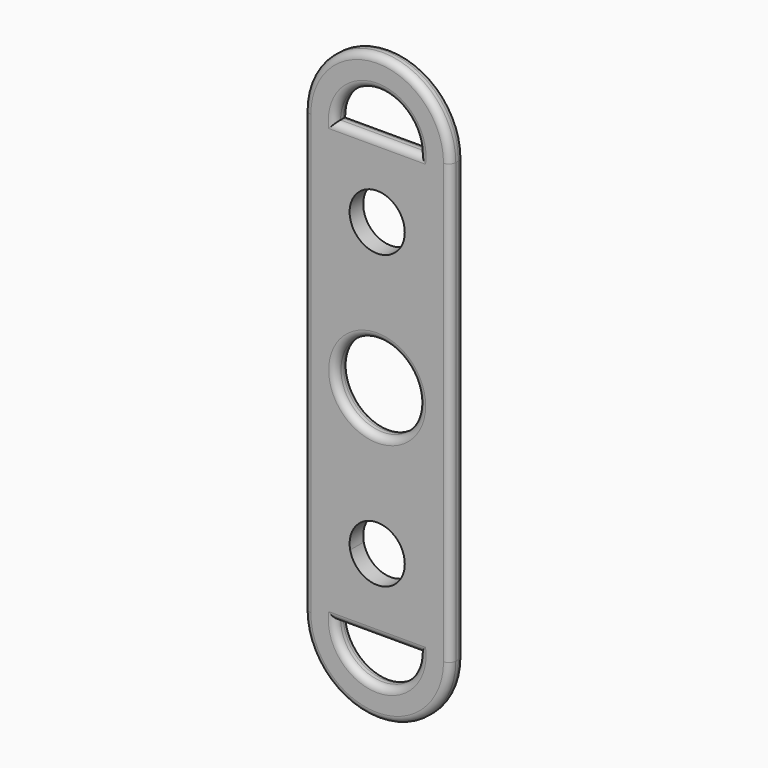
from build123d import *

# Parameters (mm, degrees)
F0_W     = 12.36
F0_H     = 4.61
F0_R     = 1
F0_R_2   = 4.05
F1_DEPTH = 2.5
F2_R     = 6.1205689933
F3_DEPTH = 25
F4_R     = 1


# Not quite as in the source:
# - a feature names something its author has since deleted; it is built from what else it names


with BuildPart() as f1:
    # F0 (on Front) → F1 (new body)
    with BuildSketch(Plane.XZ):
        with BuildLine():
            ThreePointArc((10.74, -48.33), (9.5320721777, -43.3815456959), (6.18, -39.5461967235))
            Line((6.18, -39.5461967235), (6.18, -43.72))
            Line((6.18, -43.72), (6.18, -48.33))
            ThreePointArc((6.18, -48.33), (0, -54.51), (-6.18, -48.33))
            Line((-6.18, -48.33), (-6.18, -43.72))
            Line((-6.18, -43.72), (-6.18, -39.5461967235))
            ThreePointArc((-6.18, -39.5461967235), (-9.5320721777, -43.3815456959), (-10.74, -48.33))
            ThreePointArc((-10.74, -48.33), (0, -59.07), (10.74, -48.33))
        make_face()
        with BuildLine():
            Line((6.18, 5.32), (6.18, -11.5))
            Line((6.18, -11.5), (6.18, -16.11))
            Line((6.18, -16.11), (6.18, -20.72))
            Line((6.18, -20.72), (6.18, -37.54))
            Line((6.18, -37.54), (6.18, -39.5461967235))
            ThreePointArc((6.18, -39.5461967235), (9.5320721777, -43.3815456959), (10.74, -48.33))
            Line((10.74, -48.33), (10.74, -18.9998085575))
            Line((10.74, -18.9998085575), (10.74, 16.11))
            ThreePointArc((10.74, 16.11), (0, 26.85), (-10.74, 16.11))
            Line((-10.74, 16.11), (-10.74, -18.9998085575))
            Line((-10.74, -18.9998085575), (-10.74, -48.33))
            ThreePointArc((-10.74, -48.33), (-9.5320721777, -43.3815456959), (-6.18, -39.5461967235))
            Line((-6.18, -39.5461967235), (-6.18, -37.54))
            Line((-6.18, -37.54), (-6.18, -20.72))
            Line((-6.18, -20.72), (-6.18, -16.11))
            Line((-6.18, -16.11), (-6.18, -11.5))
            Line((-6.18, -11.5), (-6.18, 5.32))
            Line((-6.18, 5.32), (-6.18, 11.5))
            Line((-6.18, 11.5), (-6.18, 16.11))
            ThreePointArc((-6.18, 16.11), (0, 22.29), (6.18, 16.11))
            Line((6.18, 16.11), (6.18, 11.5))
            Line((6.18, 11.5), (6.18, 5.32))
        make_face()
        with Locations((0, -13.805)):
            Rectangle(F0_W, F0_H)
        with Locations((0, -13.805)):
            Circle(F0_R, mode=Mode.SUBTRACT)
        with BuildLine():
            Line((-6.18, -11.5), (6.18, -11.5))
            Line((6.18, -11.5), (6.18, 5.32))
            ThreePointArc((6.18, 5.32), (0, -0.86), (-6.18, 5.32))
            Line((-6.18, 5.32), (-6.18, -11.5))
        make_face()
        with BuildLine():
            Line((6.18, -39.5461967235), (6.18, -37.54))
            ThreePointArc((6.18, -37.54), (6.1111223941, -38.4600994968), (5.9060248919, -39.3596895273))
            ThreePointArc((5.9060248919, -39.3596895273), (6.0437319312, -39.451886217), (6.18, -39.5461967235))
        make_face()
        with BuildLine():
            Line((6.18, -37.54), (6.18, -20.72))
            Line((6.18, -20.72), (-6.18, -20.72))
            Line((-6.18, -20.72), (-6.18, -37.54))
            ThreePointArc((-6.18, -37.54), (0, -31.36), (6.18, -37.54))
        make_face()
        with Locations((0, -23.415)):
            Circle(F0_R, mode=Mode.SUBTRACT)
        with BuildLine():
            Line((6.18, -43.72), (6.18, -39.5461967235))
            ThreePointArc((6.18, -39.5461967235), (6.0437319312, -39.451886217), (5.9060248919, -39.3596895273))
            ThreePointArc((5.9060248919, -39.3596895273), (4.8051050355, -41.4263048771), (3.0143614581, -42.935))
            ThreePointArc((3.0143614581, -42.935), (3.5866515341, -43.2972740217), (4.11585957, -43.72))
            Line((4.11585957, -43.72), (6.18, -43.72))
        make_face()
        with BuildLine():
            ThreePointArc((4.11585957, -43.72), (3.5866515341, -43.2972740217), (3.0143614581, -42.935))
            ThreePointArc((3.0143614581, -42.935), (1.5574498387, -43.5205309129), (0, -43.72))
            Line((0, -43.72), (4.11585957, -43.72))
        make_face()
        with BuildLine():
            Line((-6.18, -48.33), (6.18, -48.33))
            ThreePointArc((6.18, -48.33), (5.6404083249, -45.8044913525), (4.11585957, -43.72))
            Line((4.11585957, -43.72), (0, -43.72))
            Line((0, -43.72), (-4.11585957, -43.72))
            ThreePointArc((-4.11585957, -43.72), (-5.6404083249, -45.8044913525), (-6.18, -48.33))
        make_face()
        with Locations((0, -46.025)):
            Circle(F0_R, mode=Mode.SUBTRACT)
        with BuildLine():
            Line((-4.11585957, -43.72), (-6.18, -43.72))
            Line((-6.18, -43.72), (-6.18, -48.33))
            ThreePointArc((-6.18, -48.33), (-5.6404083249, -45.8044913525), (-4.11585957, -43.72))
        make_face()
        with BuildLine():
            Line((6.18, -48.33), (6.18, -43.72))
            Line((6.18, -43.72), (4.11585957, -43.72))
            ThreePointArc((4.11585957, -43.72), (5.6404083249, -45.8044913525), (6.18, -48.33))
        make_face()
        with Locations((0, -18.415)):
            Rectangle(F0_W, F0_H)
        with Locations((0, -46.025)):
            Circle(F0_R)
        with BuildLine():
            ThreePointArc((-5.9060248919, -39.3596895273), (-6.0437319312, -39.451886217), (-6.18, -39.5461967235))
            Line((-6.18, -39.5461967235), (-6.18, -43.72))
            Line((-6.18, -43.72), (-4.11585957, -43.72))
            ThreePointArc((-4.11585957, -43.72), (-3.5866515341, -43.2972740217), (-3.0143614581, -42.935))
            ThreePointArc((-3.0143614581, -42.935), (-4.8051050355, -41.4263048771), (-5.9060248919, -39.3596895273))
        make_face()
        with BuildLine():
            ThreePointArc((0, -43.72), (-1.5574498387, -43.5205309129), (-3.0143614581, -42.935))
            ThreePointArc((-3.0143614581, -42.935), (-3.5866515341, -43.2972740217), (-4.11585957, -43.72))
            Line((-4.11585957, -43.72), (0, -43.72))
        make_face()
        with BuildLine():
            ThreePointArc((5.9060248919, -39.3596895273), (6.1111223941, -38.4600994968), (6.18, -37.54))
            ThreePointArc((6.18, -37.54), (0, -31.36), (-6.18, -37.54))
            ThreePointArc((-6.18, -37.54), (-6.1111223941, -38.4600994968), (-5.9060248919, -39.3596895273))
            ThreePointArc((-5.9060248919, -39.3596895273), (-4.9628492023, -38.8054145604), (-3.9681809503, -38.3499629286))
            ThreePointArc((-3.9681809503, -38.3499629286), (-0.407042474, -33.510506679), (4.05, -37.54))
            ThreePointArc((4.05, -37.54), (4.029493321, -37.947042474), (3.9681809503, -38.3499629286))
            ThreePointArc((3.9681809503, -38.3499629286), (4.9628492023, -38.8054145604), (5.9060248919, -39.3596895273))
        make_face()
        with BuildLine():
            ThreePointArc((3.0143614581, -42.935), (4.8051050355, -41.4263048771), (5.9060248919, -39.3596895273))
            ThreePointArc((5.9060248919, -39.3596895273), (4.9628492023, -38.8054145604), (3.9681809503, -38.3499629286))
            ThreePointArc((3.9681809503, -38.3499629286), (0, -41.59), (-3.9681809503, -38.3499629286))
            ThreePointArc((-3.9681809503, -38.3499629286), (-4.9628492023, -38.8054145604), (-5.9060248919, -39.3596895273))
            ThreePointArc((-5.9060248919, -39.3596895273), (-4.8051050355, -41.4263048771), (-3.0143614581, -42.935))
            ThreePointArc((-3.0143614581, -42.935), (0, -42.15), (3.0143614581, -42.935))
        make_face()
        with BuildLine():
            ThreePointArc((0, -43.72), (1.5574498387, -43.5205309129), (3.0143614581, -42.935))
            ThreePointArc((3.0143614581, -42.935), (0, -42.15), (-3.0143614581, -42.935))
            ThreePointArc((-3.0143614581, -42.935), (-1.5574498387, -43.5205309129), (0, -43.72))
        make_face()
        with BuildLine():
            ThreePointArc((-5.9060248919, -39.3596895273), (-6.1111223941, -38.4600994968), (-6.18, -37.54))
            Line((-6.18, -37.54), (-6.18, -39.5461967235))
            ThreePointArc((-6.18, -39.5461967235), (-6.0437319312, -39.451886217), (-5.9060248919, -39.3596895273))
        make_face()
        with BuildLine():
            ThreePointArc((-6.18, 5.32), (0, -0.86), (6.18, 5.32))
            ThreePointArc((6.18, 5.32), (4.3699199077, 9.6899199077), (0, 11.5))
            ThreePointArc((0, 11.5), (-4.3699199077, 9.6899199077), (-6.18, 5.32))
        make_face()
        with Locations((0, 5.32)):
            Circle(F0_R_2, mode=Mode.SUBTRACT)
        with BuildLine():
            Line((-6.18, 11.5), (-6.18, 5.32))
            ThreePointArc((-6.18, 5.32), (-4.3699199077, 9.6899199077), (0, 11.5))
            Line((0, 11.5), (-6.18, 11.5))
        make_face()
        Polygon((0, 11.5), (6.18, 11.5), (6.18, 16.11), (-6.18, 16.11), (-6.18, 11.5), align=None)
        with Locations((0, 13.805)):
            Circle(F0_R, mode=Mode.SUBTRACT)
        with BuildLine():
            ThreePointArc((0, 11.5), (4.3699199077, 9.6899199077), (6.18, 5.32))
            Line((6.18, 5.32), (6.18, 11.5))
            Line((6.18, 11.5), (0, 11.5))
        make_face()
        with Locations((0, 13.805)):
            Circle(F0_R)
        with Locations((0, -13.805)):
            Circle(F0_R)
        with Locations((0, -23.415)):
            Circle(F0_R)
    extrude(amount=F1_DEPTH)

    # F2 (on face) → F3 (cut)
    with BuildSketch(Plane.XZ.offset(2.5)):
        with Locations((0, -16.11)):
            Circle(F2_R)
    extrude(amount=-F3_DEPTH, mode=Mode.SUBTRACT)

    # F4
    f4_edges = [f1.edges().sort_by_distance(p)[0] for p in [
        (-10.74, -2.5, -16.11),
        (0, -2.5, -54.51),
        (0, -2.5, -48.33),
        (10.74, 0, -16.11),
        (-6.120569, 0, -16.11),
        (-6.120569, -2.5, -16.11),
        (0, -2.5, 16.11),
        (0, -2.5, 22.29),
        (0, 0, 16.11),
        (0, 0, 22.29),
        (0, 0, -48.33),
        (0, 0, -54.51),
    ]]
    fillet(f4_edges, radius=F4_R)


solid = f1.part
